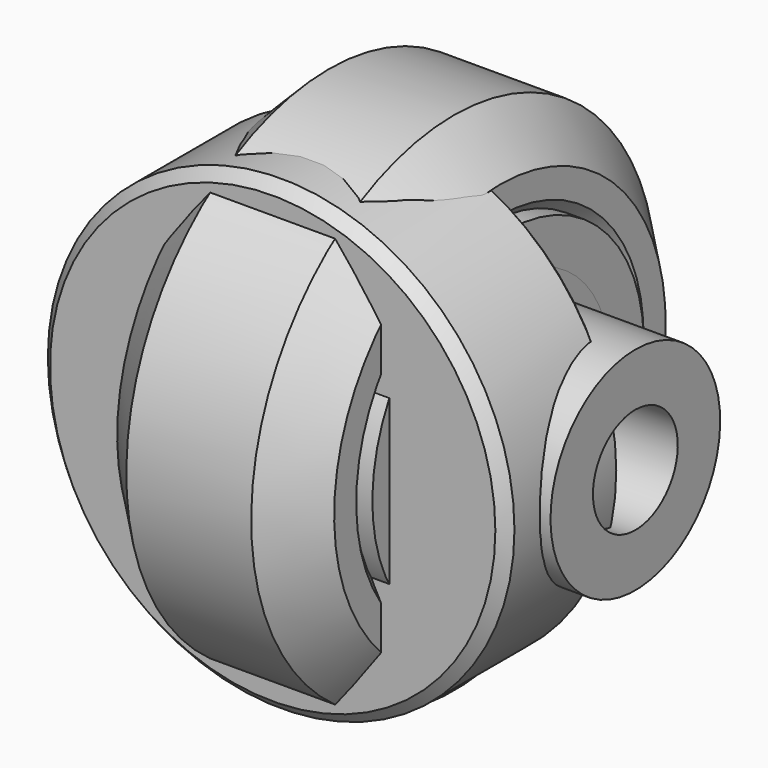
from build123d import *

# Parameters (mm, degrees)
F1_W     = 5
F1_H     = 2
F1_H_2   = 1.5
F2_W     = 6
F2_H     = 2.5
F8_R     = 11
F8_R_2   = 4
F9_DEPTH = 7
F10_SIZE = 0.5


# Not quite as in the source:
# - a feature names something its author has since deleted; it is built from what else it names


with BuildPart() as f3:
    # F0 (on Front) → F3 (revolve)
    with BuildSketch(Plane.XZ):
        Polygon((2.945, 11.945), (-2.945, 11.945), (-5.115, 9.77), (-5.115, 8.47), (-4.645, 8), (-0.5, 8), (-0.5, 7), (0.5, 7), (0.5, 8), (4.645, 8), (5.115, 8.47), (5.115, 9.77), align=None)
    revolve(axis=Axis((0.0770290499, 0, 0), (1, 0, 0)))


with BuildPart() as f4:
    # F1 (on Front) → F4 (revolve)
    with BuildSketch(Plane.XZ):
        with Locations((3, 7)):
            Rectangle(F1_W, F1_H)
    revolve(axis=Axis((0.0770290499, 0, 0), (1, 0, 0)))


with BuildPart() as f5:
    # F1 (on Front) → F5 (revolve)
    with BuildSketch(Plane.XZ):
        with Locations((3, 5.25)):
            Rectangle(F1_W, F1_H_2)
    revolve(axis=Axis((0.0770290499, 0, 0), (1, 0, 0)))


with BuildPart() as f6:
    # F1 (on Front) → F6 (revolve)
    with BuildSketch(Plane.XZ):
        with Locations((3, 3.5)):
            Rectangle(F1_W, F1_H)
    revolve(axis=Axis((0.0770290499, 0, 0), (1, 0, 0)))


with BuildPart() as f7:
    # F2 (on Front) → F7 (revolve)
    with BuildSketch(Plane.XZ):
        with Locations((8.5, 3.75)):
            Rectangle(F2_W, F2_H)
    revolve(axis=Axis((0.0770290499, 0, 0), (1, 0, 0)))


with BuildPart() as f9:
    # F8 (on Front) → F9 (new body)
    with BuildSketch(Plane.XZ):
        Circle(F8_R)
        Circle(F8_R_2, mode=Mode.SUBTRACT)
    extrude(amount=F9_DEPTH)

    # F10
    f10_edges = [f9.edges().sort_by_distance(p)[0] for p in [
        (-11, -7, 0),
        (-11, 0, 0),
    ]]
    chamfer(f10_edges, length=F10_SIZE)


solid = Compound([f3.part, f4.part, f5.part, f6.part, f7.part, f9.part])
